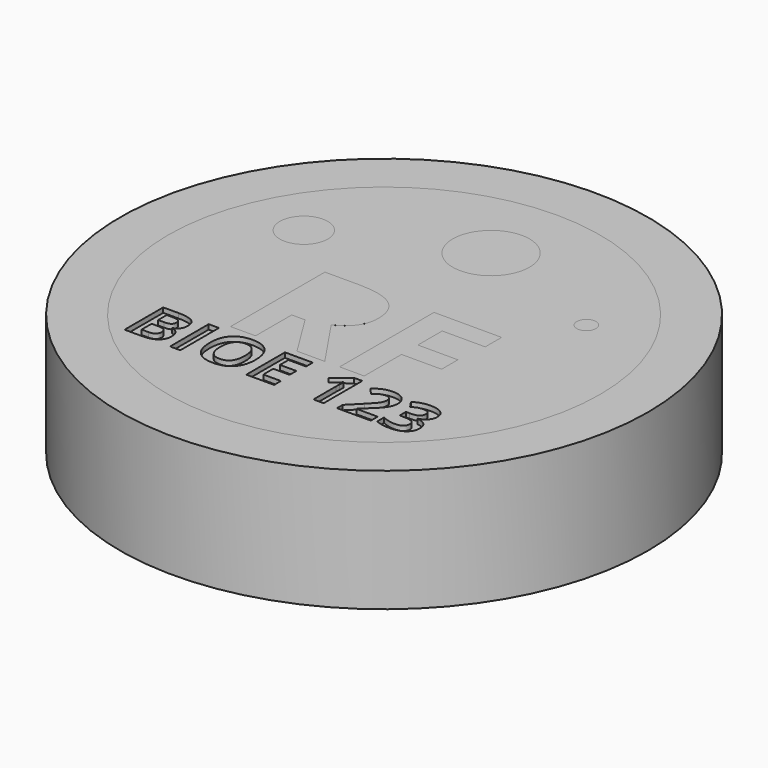
from build123d import *

# Parameters (mm, degrees)
F0_R         = 4
F0_TEXT_SIZE = 17.2183591834
F0_R_2       = 2.5
F0_R_3       = 1
F1_DEPTH     = 12.7
F0_R_4       = 27.5
F0_R_5       = 22.5
F2_DEPTH     = 12.7
F3_DEPTH     = 6.35
F4_DEPTH     = 6.35
F5_TEXT_SIZE = 7.0493228527
F6_DEPTH     = 0.5


# Not quite as in the source:
# - a feature names something its author has since deleted; it is built from what else it names
# - Text() gives the source's letters only with a copy of the font that has no kerning and outlines rounded to 1/6400 em; it was checked with that copy


with BuildPart() as f1:
    # F0 (on Top) → F1 (new body)
    with BuildSketch(Plane.XY):
        with Locations((0.0112405126, 13.9230438331)):
            Circle(F0_R)
        with Locations((-9.9980669329, -9.4362896634)):
            Text('RF', F0_TEXT_SIZE, font='Open Sans', font_style=FontStyle.BOLD, text_align=(TextAlign.LEFT, TextAlign.BOTTOM))
        with Locations((-14.4008066475, 7.5470063301)):
            Circle(F0_R_2)
        with BuildLine():
            Line((-5.8441377799, 0.7198518861), (-5.8441377799, -2.6000629939))
            Line((-5.8441377799, -2.6000629939), (-5.0047427697, -2.6000629939))
            add(Edge.make_bspline(
                [(-5.0047427697, -2.6000629939), (-3.7671732034, -2.6000629939), (-3.1793276594, -2.1884365947)],
                knots=[0, 0, 0, 1, 1, 1], degree=2))
            add(Edge.make_bspline(
                [(-3.1793276594, -2.1884365947), (-2.5914821154, -1.7768101955), (-2.5914821154, -0.8943692873)],
                knots=[0, 0, 0, 1, 1, 1], degree=2))
            add(Edge.make_bspline(
                [(-2.5914821154, -0.8943692873), (-2.5914821154, -0.019999485), (-3.1927795025, 0.3499262006)],
                knots=[0, 0, 0, 1, 1, 1], degree=2))
            add(Edge.make_bspline(
                [(-3.1927795025, 0.3499262006), (-3.7940768896, 0.7198518861), (-5.0531694049, 0.7198518861)],
                knots=[0, 0, 0, 1, 1, 1], degree=2))
            Line((-5.0531694049, 0.7198518861), (-5.8441377799, 0.7198518861))
        make_face()
        with Locations((13.9879078749, 8.8628650396)):
            Circle(F0_R_3)
    extrude(amount=F1_DEPTH)



with BuildPart() as f2:
    # F0 (on Top) → F2 (new body)
    with BuildSketch(Plane.XY):
        Circle(F0_R_4)
        Circle(F0_R_5, mode=Mode.SUBTRACT)
    extrude(amount=F2_DEPTH)


with BuildPart() as f1_1:
    add(f1.part)

    add(f2.part)  # F3 merges F2
    # F0 (on Top) → F3 (join)
    with BuildSketch(Plane.XY):
        Circle(F0_R_5)
        with BuildLine():
            Line((-4.4585979394, -4.7200734684), (-5.8441377799, -4.7200734684))
            Line((-5.8441377799, -4.7200734684), (-5.8441377799, -9.4362896634))
            Line((-5.8441377799, -9.4362896634), (-8.451104975, -9.4362896634))
            Line((-8.451104975, -9.4362896634), (-8.451104975, 2.8560045723))
            Line((-8.451104975, 2.8560045723), (-4.8702243386, 2.8560045723))
            add(Edge.make_bspline(
                [(-4.8702243386, 2.8560045723), (-2.3628007825, 2.8560045723), (-1.1615511926, 1.9439696093)],
                knots=[0, 0, 0, 1, 1, 1], degree=2))
            add(Edge.make_bspline(
                [(-1.1615511926, 1.9439696093), (0.0396983973, 1.0319346463), (0.0396983973, -0.8271100717)],
                knots=[0, 0, 0, 1, 1, 1], degree=2))
            add(Edge.make_bspline(
                [(0.0396983973, -0.8271100717), (0.0396983973, -1.9113286266), (-0.5562182526, -2.756104374)],
                knots=[0, 0, 0, 1, 1, 1], degree=2))
            add(Edge.make_bspline(
                [(-0.5562182526, -2.756104374), (-1.1521349024, -3.6008801214), (-2.2471149318, -4.0797657362)],
                knots=[0, 0, 0, 1, 1, 1], degree=2))
            add(Edge.make_bspline(
                [(-2.2471149318, -4.0797657362), (0.5293454866, -8.2256237833), (1.3687404967, -9.4362896634)],
                knots=[0, 0, 0, 1, 1, 1], degree=2))
            Line((1.3687404967, -9.4362896634), (-1.5234057723, -9.4362896634))
            Line((-1.5234057723, -9.4362896634), (-4.4585979394, -4.7200734684))
        make_face(mode=Mode.SUBTRACT)
        Polygon((5.4796237518, -4.5774839314), (5.4796237518, -9.4362896634), (2.9157024546, -9.4362896634), (2.9157024546, 2.8560045723), (9.9617778767, 2.8560045723), (9.9617778767, 0.7198518861), (5.4796237518, 0.7198518861), (5.4796237518, -2.4494023511), (9.6496951165, -2.4494023511), (9.6496951165, -4.5774839314), align=None, mode=Mode.SUBTRACT)
        with Locations((-14.4008066475, 7.5470063301)):
            Circle(F0_R_2, mode=Mode.SUBTRACT)
        with Locations((13.9879078749, 8.8628650396)):
            Circle(F0_R_3, mode=Mode.SUBTRACT)
        with Locations((0.0112405126, 13.9230438331)):
            Circle(F0_R, mode=Mode.SUBTRACT)
    extrude(amount=F3_DEPTH)


with BuildPart() as f4:
    # F4 (new): a face of the model
    f4_faces = [f1_1.part.faces().sort_by_distance(p)[0] for p in [
        (0.2438445214, -0.3793024692, 6.35),
    ]]
    extrude(f4_faces, amount=F4_DEPTH)

    # F5 (on face) → F6 (cut)
    with BuildSketch(Plane.XY.offset(12.7)):
        with Locations((-15.4738517012, -15.2455922216)):
            Text('BIOE 123', F5_TEXT_SIZE, font='Open Sans', font_style=FontStyle.BOLD, text_align=(TextAlign.LEFT, TextAlign.BOTTOM))
    extrude(amount=-F6_DEPTH, mode=Mode.SUBTRACT)


solid = Compound([f1_1.part, f4.part])
